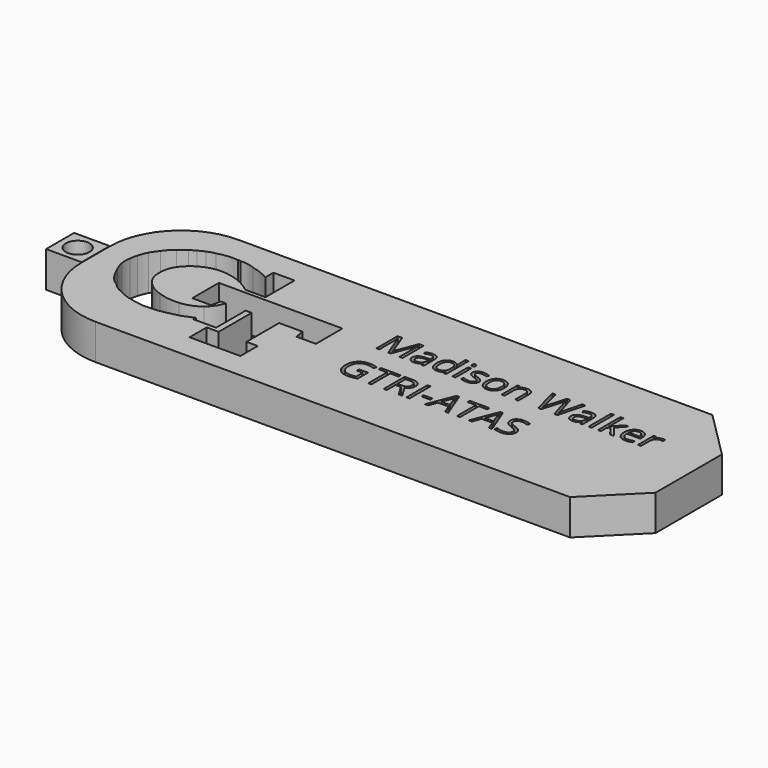
from build123d import *

# Parameters (mm, degrees)
F0_W         = 63.5
F0_H         = 19.05
F1_DEPTH     = 3.81
F3_DEPTH     = 3.81
F4_SIZE      = 5.08
F5_R         = 7.62
F6_TEXT_SIZE = 3.9496240571
F7_DEPTH     = 2.54
F8_W         = 3.7519996986
F8_H         = 3.8419382181
F9_DEPTH     = 3.81
F10_R        = 1.27
F11_DEPTH    = 5080


# Not quite as in the source:
# - Text() gives the source's letters only with a copy of the font that has no kerning and outlines rounded to 1/6400 em; it was checked with that copy


with BuildPart() as f1:
    # F0 (on Top) → F1 (new body)
    with BuildSketch(Plane.XY):
        with Locations((31.75, 9.525)):
            Rectangle(F0_W, F0_H)
    extrude(amount=F1_DEPTH)

    # F2 (on face) → F3 (cut)
    with BuildSketch(Plane.XY.offset(3.81)):
        with BuildLine():
            ThreePointArc((10.0632179528, 13.7286745012), (12.0302600212, 13.3564931218), (13.7608833611, 12.3501550406))
            Line((13.7608833611, 12.3501550406), (15.9242320806, 12.3501550406))
            Line((15.9242320806, 12.3501550406), (15.9242320806, 16.230661422))
            Line((15.9242320806, 16.230661422), (13.6662377045, 16.230661422))
            Line((13.6662377045, 16.230661422), (13.6662377045, 15.148986131))
            ThreePointArc((13.6662377045, 15.148986131), (12.7471646405, 15.5905367404), (11.7733078077, 15.8926378936))
            ThreePointArc((11.7733078077, 15.8926378936), (10.9908090025, 16.1177383644), (10.1778386161, 16.1630567163))
            ThreePointArc((10.1778386161, 16.1630567163), (10.0426292047, 16.2036195397), (9.9074197933, 16.1630567163))
            ThreePointArc((9.9074197933, 16.1630567163), (8.8148721247, 16.1776364364), (7.7440720052, 15.9602425992))
            ThreePointArc((7.7440720052, 15.9602425992), (7.2995838936, 15.8716031678), (6.8787327036, 15.7033447176))
            ThreePointArc((6.8787327036, 15.7033447176), (6.5259731416, 15.5506045404), (6.1891656369, 15.3653221205))
            ThreePointArc((6.1891656369, 15.3653221205), (5.8630266549, 15.19331237), (5.5672032759, 14.9732157588))
            ThreePointArc((5.5672032759, 14.9732157588), (5.1458196364, 14.6952764268), (4.7424267977, 14.3918152899))
            ThreePointArc((4.7424267977, 14.3918152899), (4.2473377596, 13.9240499895), (3.8230037317, 13.3912665769))
            ThreePointArc((3.8230037317, 13.3912665769), (3.5130015264, 12.9785319205), (3.2416037284, 12.5394482166))
            ThreePointArc((3.2416037284, 12.5394482166), (3.0180195087, 12.0499634719), (2.8494971339, 11.538900435))
            ThreePointArc((2.8494971339, 11.538900435), (2.7563041075, 11.1356861253), (2.6872456074, 10.727644898))
            ThreePointArc((2.6872456074, 10.727644898), (2.643848535, 10.1935681887), (2.6872456074, 9.6594914794))
            ThreePointArc((2.6872456074, 9.6594914794), (2.8303599919, 9.1251141932), (3.0523107853, 8.6183808744))
            ThreePointArc((3.0523107853, 8.6183808744), (3.3247118474, 8.0411344978), (3.6337107886, 7.4826227501))
            ThreePointArc((3.6337107886, 7.4826227501), (4.1213107787, 6.8674431298), (4.7424267977, 6.3874279149))
            ThreePointArc((4.7424267977, 6.3874279149), (5.2209227876, 5.9567191408), (5.7835378684, 5.6437770836))
            ThreePointArc((5.7835378684, 5.6437770836), (6.4661904627, 5.3228890448), (7.1832598187, 5.088805221))
            ThreePointArc((7.1832598187, 5.088805221), (7.9288828181, 4.9215247247), (8.6840828881, 4.8048659228))
            ThreePointArc((8.6840828881, 4.8048659228), (9.1437939554, 4.7723975943), (9.6035050228, 4.8048659228))
            ThreePointArc((9.6035050228, 4.8048659228), (10.2015105721, 4.8355496003), (10.7933469117, 4.926554393))
            ThreePointArc((10.7933469117, 4.926554393), (11.6617822056, 5.101694226), (12.5240255147, 5.3051402792))
            ThreePointArc((12.5240255147, 5.3051402792), (13.1135497518, 5.5520696782), (13.7003455311, 5.8054146357))
            Line((13.7003455311, 5.8054146357), (13.7003455311, 5.4673915729))
            Line((13.7003455311, 5.4673915729), (16.1476340145, 5.4673915729))
            Line((16.1476340145, 5.4673915729), (16.1476340145, 9.4155017287))
            Line((16.1476340145, 9.4155017287), (16.7831163853, 9.4155017287))
            Line((16.7831163853, 9.4155017287), (16.7831163853, 5.0076800399))
            Line((16.7831163853, 5.0076800399), (15.4986288399, 5.0076800399))
            Line((15.4986288399, 5.0076800399), (15.4986288399, 2.7226433158))
            Line((15.4986288399, 2.7226433158), (20.9340397269, 2.7226433158))
            Line((20.9340397269, 2.7226433158), (20.9340397269, 5.0482423976))
            Line((20.9340397269, 5.0482423976), (19.7306796908, 5.0482423976))
            Line((19.7306796908, 5.0482423976), (19.7306796908, 9.4155017287))
            Line((19.7306796908, 9.4155017287), (22.218529135, 9.4155017287))
            Line((22.218529135, 9.4155017287), (22.4213432521, 8.3879111335))
            Line((22.4213432521, 8.3879111335), (24.4900435209, 8.3879111335))
            Line((24.4900435209, 8.3879111335), (24.4900435209, 11.9439139962))
            Line((24.4900435209, 11.9439139962), (15.7014429569, 11.9439139962))
            Line((15.7014429569, 11.9439139962), (11.2530589104, 11.9439139962))
            Line((11.2530589104, 11.9439139962), (11.2530589104, 8.3879111335))
            Line((11.2530589104, 8.3879111335), (13.2676772773, 8.3879111335))
            Line((13.2676772773, 8.3879111335), (13.4840123355, 9.4155017287))
            Line((13.4840123355, 9.4155017287), (14.0383699909, 9.4155017287))
            ThreePointArc((14.0383699909, 9.4155017287), (13.6055461429, 8.5383917888), (12.9566956311, 7.8065097332))
            ThreePointArc((12.9566956311, 7.8065097332), (11.9854383533, 7.2750204122), (10.9015153721, 7.0493379608))
            ThreePointArc((10.9015153721, 7.0493379608), (9.7575422741, 7.0722138489), (8.643520996, 7.3332777247))
            ThreePointArc((8.643520996, 7.3332777247), (7.6129638073, 7.8171551203), (6.7776329815, 8.5907233879))
            ThreePointArc((6.7776329815, 8.5907233879), (6.3680437853, 9.3066129529), (6.2232753262, 10.1185878739))
            ThreePointArc((6.2232753262, 10.1185878739), (6.3634108937, 11.2626407259), (6.9263633341, 12.2684137896))
            ThreePointArc((6.9263633341, 12.2684137896), (8.3434406216, 13.3236662357), (10.0632179528, 13.7286745012))
        make_face()
    extrude(amount=-F3_DEPTH, mode=Mode.SUBTRACT)

    # F4
    f4_edges = [f1.edges().sort_by_distance(p)[0] for p in [
        (63.5, 0, 1.905),
        (63.5, 19.05, 1.905),
    ]]
    chamfer(f4_edges, length=F4_SIZE)

    # F5
    f5_edges = [f1.edges().sort_by_distance(p)[0] for p in [
        (0, 0, 1.905),
        (0, 19.05, 1.905),
    ]]
    fillet(f5_edges, radius=F5_R)

    # F6 (on face) → F7 (cut)
    with BuildSketch(Plane.XY.offset(3.81)):
        with Locations((28.5645449009, 10.9230706789)):
            Text('Madison Walker', F6_TEXT_SIZE, font='Open Sans', text_align=(TextAlign.LEFT, TextAlign.BOTTOM))
        with Locations((28.5645449009, 5.5515819612)):
            Text('GTRI-ATAS', F6_TEXT_SIZE, font='Open Sans', text_align=(TextAlign.LEFT, TextAlign.BOTTOM))
    extrude(amount=-F7_DEPTH, mode=Mode.SUBTRACT)

    # F8 (on Right) → F9 (join)
    with BuildSketch(Plane.YZ):
        with Locations((9.526330512, 1.9209691091)):
            Rectangle(F8_W, F8_H)
    extrude(amount=-F9_DEPTH)

    # F10 (on face) → F11 (cut)
    with BuildSketch(Plane.XY.offset(3.8419382181)):
        with Locations((-1.905, 9.4973303613)):
            Circle(F10_R)
    extrude(amount=-F11_DEPTH, mode=Mode.SUBTRACT)


solid = f1.part
